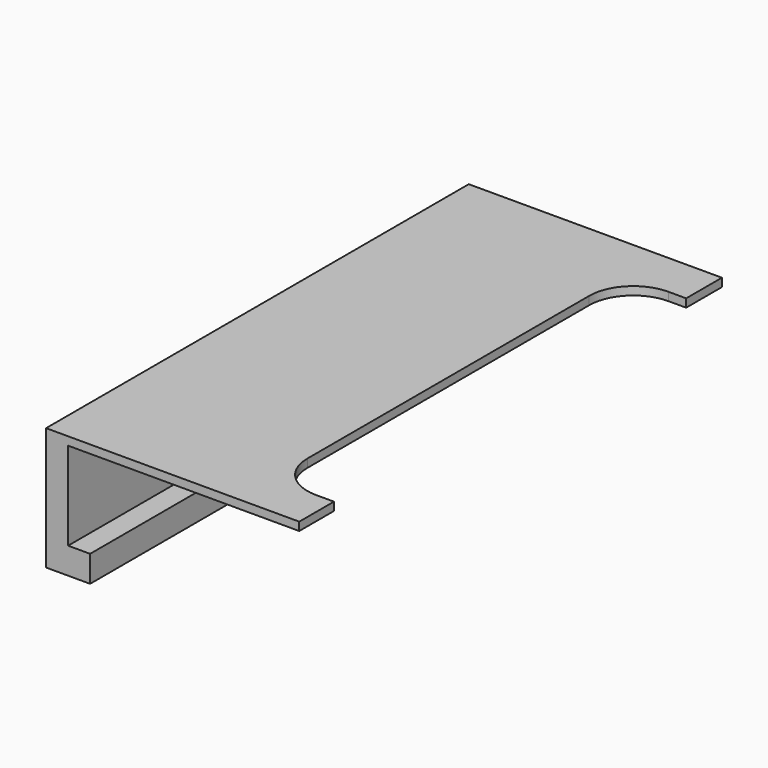
from build123d import *

# Parameters (mm, degrees)
F0_W     = 3.175
F0_H     = 76.2
F1_DEPTH = 1.190625
F2_DEPTH = 16.51
F3_START = -12.7
F3_DEPTH = 3.81


# Not quite as in the source:
# - a length typed as a fraction of an inch, garbled in the dataset ("3 / 203.2 mm" for 3/8 in), is restored


with BuildPart() as f1:
    # F0 (on Top) → F1 (new body)
    with BuildSketch(Plane.XY):
        with Locations((-34.925, 0)):
            Rectangle(F0_W, F0_H)
        with BuildLine():
            Line((-30.1625, 38.1), (-30.1625, -38.1))
            Line((-30.1625, -38.1), (0, -38.1))
            Line((0, -38.1), (0, -31.8450108171))
            Line((0, -31.8450108171), (-2.553815411, -31.8450108171))
            ThreePointArc((-2.553815411, -31.8450108171), (-7.0439434716, -29.9851388776), (-8.903815411, -25.4950108171))
            Line((-8.903815411, -25.4950108171), (-8.903815411, 25.3049891829))
            ThreePointArc((-8.903815411, 25.3049891829), (-7.0439434716, 29.7951172435), (-2.553815411, 31.6549891829))
            Line((-2.553815411, 31.6549891829), (0, 31.6549891829))
            Line((0, 31.6549891829), (0, 38.1))
            Line((0, 38.1), (-30.1625, 38.1))
        make_face()
        with Locations((-31.75, 0)):
            Rectangle(F0_W, F0_H)
    extrude(amount=F1_DEPTH)

    # F0 (on Top) → F2 (join)
    with BuildSketch(Plane.XY):
        with Locations((-34.925, 0)):
            Rectangle(F0_W, F0_H)
    extrude(amount=-F2_DEPTH)

    # F0 (on Top) → F3 (join)
    with BuildSketch(Plane.XY.offset(F3_START)):
        with Locations((-34.925, 0)):
            Rectangle(F0_W, F0_H)
        with Locations((-31.75, 0)):
            Rectangle(F0_W, F0_H)
    extrude(amount=-F3_DEPTH)


solid = f1.part
